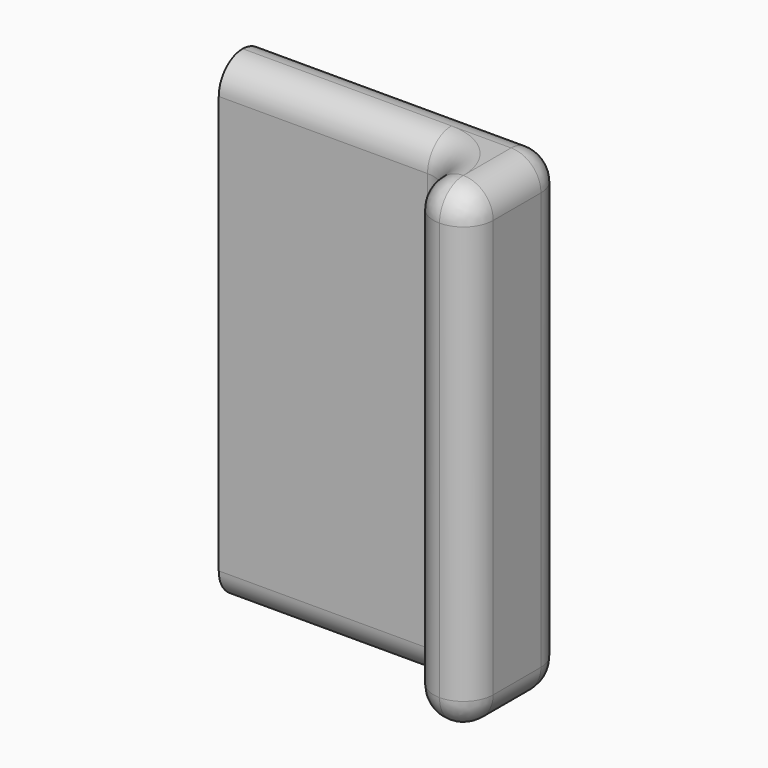
from build123d import *

# Parameters (mm, degrees)
F0_W         = 25.4
F0_H         = 50.8
F0_W_2       = 6.35
F1_DEPTH     = 6.35
F2_DEPTH     = 12.7
F3_R         = 3.17499
F4_T1_DEPTH  = 30.16251
F4_T3_DEPTH  = 44.45001
F4_T5_DEPTH  = 17.46251
F4_T7_DEPTH  = 3.17501
F4_T10_ANGLE = 90
F4_T12_ANGLE = 90
F4_T14_ANGLE = 90
F4_T16_ANGLE = 90
F4_T18_ANGLE = 90
F4_T20_ANGLE = 90
F4_T22_ANGLE = 90
F4_T24_ANGLE = 90


# Not quite as in the source:
# - a fillet or chamfer that OpenCascade refuses, or shapes differently, is made with other operations: its cross-section is extruded or revolved along the edge and cut away or added
# - a fillet or chamfer is up to 0.001 mm smaller than in the source, because OpenCascade refuses the exact size


with BuildPart() as f1:
    # F0 (on Front) → F1 (new body)
    with BuildSketch(Plane.XZ):
        with Locations((-19.05, 25.4)):
            Rectangle(F0_W, F0_H)
        with Locations((-3.175, 25.4)):
            Rectangle(F0_W_2, F0_H)
    extrude(amount=F1_DEPTH)

    # F0 (on Front) → F2 (join)
    with BuildSketch(Plane.XZ):
        with Locations((-3.175, 25.4)):
            Rectangle(F0_W_2, F0_H)
    extrude(amount=F2_DEPTH)

    # F3 (radius 3.175 in the source; OpenCascade refuses exactly that, so slightly less here)
    f3_edges = [f1.edges().sort_by_distance(p)[0] for p in [
        (0, 0, 25.4),
        (-6.35, -6.35, 25.4),
        (-3.175, -12.7, 0),
        (0, -12.7, 25.4),
        (-3.175, -12.7, 50.8),
        (-6.35, -12.7, 25.4),
    ]]
    fillet(f3_edges, radius=F3_R)

    # F4: fillet of radius 3.175 on 4 edges, made by hand

    # F4_s2 → F4_t1 (cut)
    with BuildSketch(Plane.YZ.offset(-39.6875)):
        with BuildLine():
            ThreePointArc((-6.35, 47.625), (-5.4200640303, 49.8700640303), (-3.175, 50.8))
            Line((-3.175, 50.8), (-6.35, 50.8))
            Line((-6.35, 50.8), (-6.35, 47.625))
        make_face()
        with BuildLine():
            ThreePointArc((-6.35, 3.175), (-5.4200640303, 0.9299359697), (-3.175, 0))
            Line((-3.175, 0), (-6.35, 0))
            Line((-6.35, 0), (-6.35, 3.175))
        make_face()
    extrude(amount=F4_T1_DEPTH, mode=Mode.SUBTRACT)

    # F4_s4 → F4_t3 (cut)
    with BuildSketch(Plane.YZ.offset(-39.6875)):
        with BuildLine():
            ThreePointArc((-3.175, 0), (-0.9299359697, 0.9299359697), (0, 3.175))
            Line((0, 3.175), (0, 0))
            Line((0, 0), (-3.175, 0))
        make_face()
        with BuildLine():
            ThreePointArc((-3.175, 50.8), (-0.9299359697, 49.8700640303), (0, 47.625))
            Line((0, 47.625), (0, 50.8))
            Line((0, 50.8), (-3.175, 50.8))
        make_face()
    extrude(amount=F4_T3_DEPTH, mode=Mode.SUBTRACT)

    # F4_s6 → F4_t5 (cut)
    with BuildSketch(Plane.XZ.offset(-4.76251)):
        with BuildLine():
            ThreePointArc((-3.175, 50.8), (-0.9299359697, 49.8700640303), (0, 47.625))
            Line((0, 47.625), (0, 50.8))
            Line((0, 50.8), (-3.175, 50.8))
        make_face()
        with BuildLine():
            ThreePointArc((-3.175, 0), (-0.9299359697, 0.9299359697), (0, 3.175))
            Line((0, 3.175), (0, 0))
            Line((0, 0), (-3.175, 0))
        make_face()
    extrude(amount=F4_T5_DEPTH, mode=Mode.SUBTRACT)

    # F4_s8 → F4_t7 (cut)
    with BuildSketch(Plane.XZ.offset(9.52499)):
        with BuildLine():
            ThreePointArc((-3.175, 0), (-5.4200640303, 0.9299359697), (-6.35, 3.175))
            Line((-6.35, 3.175), (-6.35, 0))
            Line((-6.35, 0), (-3.175, 0))
        make_face()
        with BuildLine():
            ThreePointArc((-3.175, 50.8), (-5.4200640303, 49.8700640303), (-6.35, 47.625))
            Line((-6.35, 47.625), (-6.35, 50.8))
            Line((-6.35, 50.8), (-3.175, 50.8))
        make_face()
    extrude(amount=F4_T7_DEPTH, mode=Mode.SUBTRACT)

    # F4_s9 → F4_t10 (revolve, cut)
    with BuildSketch(Plane.XY.offset(47.625)):
        with BuildLine():
            ThreePointArc((-3.17499, -12.7), (-0.9299330408, -11.7700669592), (0, -9.52501))
            Line((0, -9.52501), (0, -12.7))
            Line((0, -12.7), (-3.17499, -12.7))
        make_face()
    revolve(axis=Axis((-3.175, -12.7, 47.625), (0, -1, 0)), revolution_arc=F4_T10_ANGLE, mode=Mode.SUBTRACT)

    # F4_s11 → F4_t12 (revolve, cut)
    with BuildSketch(Plane.YZ.offset(-3.175)):
        with BuildLine():
            ThreePointArc((-12.7, 3.17499), (-11.7700669592, 0.9299330408), (-9.52501, 0))
            Line((-9.52501, 0), (-12.7, 0))
            Line((-12.7, 0), (-12.7, 3.17499))
        make_face()
    revolve(axis=Axis((-3.175, -12.7, 3.175), (0, -1, 0)), revolution_arc=F4_T12_ANGLE, mode=Mode.SUBTRACT)

    # F4_s13 → F4_t14 (revolve, cut)
    with BuildSketch(Plane.XY.offset(3.175)):
        with BuildLine():
            ThreePointArc((-3.17501, -12.7), (-5.4200669592, -11.7700669592), (-6.35, -9.52501))
            Line((-6.35, -9.52501), (-6.35, -12.7))
            Line((-6.35, -12.7), (-3.17501, -12.7))
        make_face()
    revolve(axis=Axis((-3.175, -12.7, 3.175), (0, -1, 0)), revolution_arc=F4_T14_ANGLE, mode=Mode.SUBTRACT)

    # F4_s15 → F4_t16 (revolve, cut)
    with BuildSketch(Plane.YZ.offset(-3.175)):
        with BuildLine():
            ThreePointArc((-12.7, 47.62501), (-11.7700669592, 49.8700669592), (-9.52501, 50.8))
            Line((-9.52501, 50.8), (-12.7, 50.8))
            Line((-12.7, 50.8), (-12.7, 47.62501))
        make_face()
    revolve(axis=Axis((-3.175, -12.7, 47.625), (0, -1, 0)), revolution_arc=F4_T16_ANGLE, mode=Mode.SUBTRACT)

    # F4_s17 → F4_t18 (revolve, cut)
    with BuildSketch(Plane.XZ.offset(3.17499)):
        with BuildLine():
            ThreePointArc((-3.17499, 50.8), (-0.9299324342, 49.8700604947), (0, 47.625))
            Line((0, 47.625), (0, 50.8))
            Line((0, 50.8), (-3.17499, 50.8))
        make_face()
    revolve(axis=Axis((-3.17499, -3.17499, 50.8), (0, 0, 1)), revolution_arc=F4_T18_ANGLE, mode=Mode.SUBTRACT)

    # F4_s19 → F4_t20 (revolve, cut)
    with BuildSketch(Plane.XZ.offset(3.17499)):
        with BuildLine():
            ThreePointArc((-3.17499, 0), (-0.9299324342, 0.9299395053), (0, 3.175))
            Line((0, 3.175), (0, 0))
            Line((0, 0), (-3.17499, 0))
        make_face()
    revolve(axis=Axis((-3.17499, -3.17499, 0), (0, 0, 1)), revolution_arc=F4_T20_ANGLE, mode=Mode.SUBTRACT)

    # F4_s21 → F4_t22 (revolve, cut)
    with BuildSketch(Plane.YZ.offset(-9.52499)):
        with BuildLine():
            ThreePointArc((-6.35, 3.175), (-5.4200640303, 0.9299359697), (-3.175, 0))
            Line((-3.175, 0), (-6.35, 0))
            Line((-6.35, 0), (-6.35, 3.175))
        make_face()
    revolve(axis=Axis((-9.52499, -9.52499, 0), (0, 0, -1)), revolution_arc=F4_T22_ANGLE, mode=Mode.SUBTRACT)

    # F4_s23 → F4_t24 (revolve, cut)
    with BuildSketch(Plane.YZ.offset(-9.52499)):
        with BuildLine():
            ThreePointArc((-3.175, 50.8), (-5.4200640303, 49.8700640303), (-6.35, 47.625))
            Line((-6.35, 47.625), (-6.35, 50.8))
            Line((-6.35, 50.8), (-3.175, 50.8))
        make_face()
    revolve(axis=Axis((-9.52499, -9.52499, 50.8), (0, 0, -1)), revolution_arc=F4_T24_ANGLE, mode=Mode.SUBTRACT)


solid = f1.part
